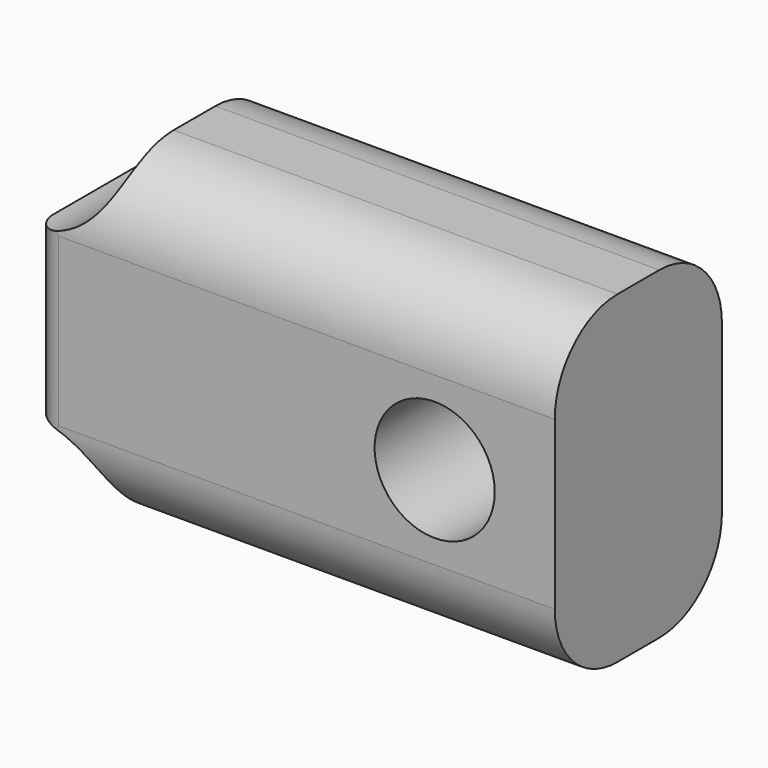
from build123d import *

# Parameters (mm, degrees)
F0_R        = 1.15
F1_DEPTH    = 4
F2_R        = 1.5
F3_DEPTH    = 5
F4_T1_DEPTH = 16
F5_R        = 0.49999


# Not quite as in the source:
# - a fillet or chamfer that OpenCascade refuses, or shapes differently, is made with other operations: its cross-section is extruded or revolved along the edge and cut away or added
# - a fillet or chamfer is up to 0.001 mm smaller than in the source, because OpenCascade refuses the exact size


with BuildPart() as f1:
    # F0 (on Front) → F1 (new body)
    with BuildSketch(Plane.XZ):
        with BuildLine():
            Line((-3.5, -3.1), (5, -3.1))
            Line((5, -3.1), (5, 3.1))
            Line((5, 3.1), (-3.5, 3.1))
            ThreePointArc((-3.5, 3.1), (-3.9393398282, 2.0393398282), (-5, 1.6))
            Line((-5, 1.6), (-5, -1.6))
            ThreePointArc((-5, -1.6), (-3.9393398282, -2.0393398282), (-3.5, -3.1))
        make_face()
        with Locations((2.7, 0)):
            Circle(F0_R, mode=Mode.SUBTRACT)
    extrude(amount=F1_DEPTH)

    # F2 (on face) → F3 (cut)
    with BuildSketch(Plane(origin=(-5, 0, 0), x_dir=(0, -1, 0), z_dir=(-1, 0, 0))):
        with Locations((2, 0)):
            Circle(F2_R)
    extrude(amount=-F3_DEPTH, mode=Mode.SUBTRACT)

    # F4: fillet of radius 1.5 on 4 edges, made by hand

    # F4_s2 → F4_t1 (cut)
    with BuildSketch(Plane.YZ.offset(-7.25)):
        with BuildLine():
            ThreePointArc((0, 1.6), (-0.4393398282, 2.6606601718), (-1.5, 3.1))
            Line((-1.5, 3.1), (0, 3.1))
            Line((0, 3.1), (0, 1.6))
        make_face()
        with BuildLine():
            ThreePointArc((-4, 1.6), (-3.5606601718, 2.6606601718), (-2.5, 3.1))
            Line((-2.5, 3.1), (-4, 3.1))
            Line((-4, 3.1), (-4, 1.6))
        make_face()
        with BuildLine():
            ThreePointArc((-2.5, -3.1), (-3.5606601718, -2.6606601718), (-4, -1.6))
            Line((-4, -1.6), (-4, -3.1))
            Line((-4, -3.1), (-2.5, -3.1))
        make_face()
        with BuildLine():
            ThreePointArc((-1.5, -3.1), (-0.4393398282, -2.6606601718), (0, -1.6))
            Line((0, -1.6), (0, -3.1))
            Line((0, -3.1), (-1.5, -3.1))
        make_face()
    extrude(amount=F4_T1_DEPTH, mode=Mode.SUBTRACT)

    # F5 (radius 0.5 in the source; OpenCascade refuses exactly that, so slightly less here)
    f5_edges = [f1.edges().sort_by_distance(p)[0] for p in [
        (-5, 0, 0),
        (-5, -4, 0),
    ]]
    fillet(f5_edges, radius=F5_R)


solid = f1.part
